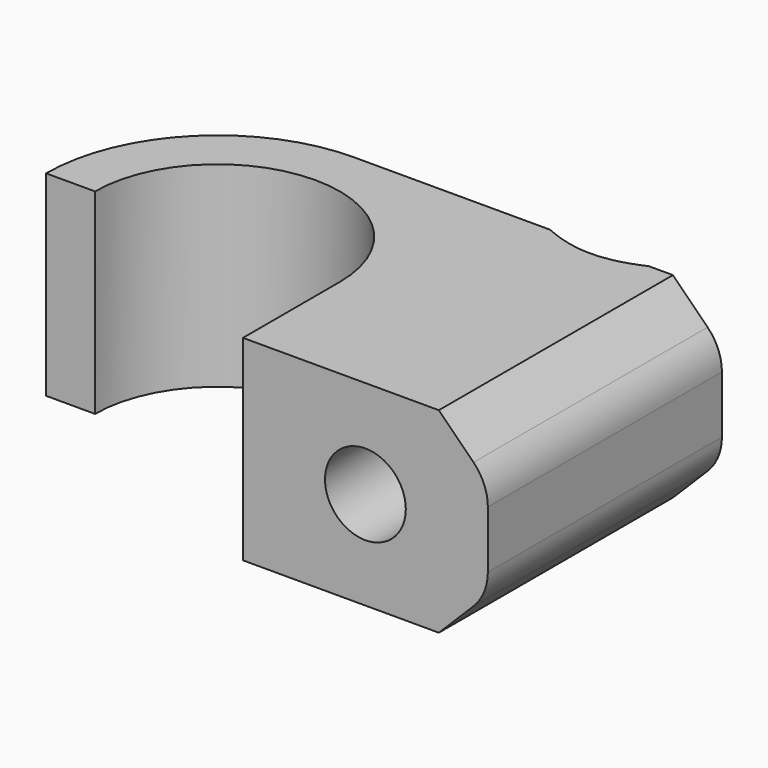
from build123d import *

# Parameters (mm, degrees)
F1_DEPTH       = 4
F3_D           = 3.3
F3_CSINK_D     = 8.96
F3_CSINK_ANGLE = 90
F4_SIZE        = 2
F5_R           = 2


with BuildPart() as f1:
    # F0 (on Top) → F1 (new body, symmetric)
    with BuildSketch(Plane.XY):
        with BuildLine():
            ThreePointArc((-53.8887429237, 51.9443377852), (-48.8887429237, 56.9443377852), (-43.8887429237, 51.9443377852))
            Line((-43.8887429237, 51.9443377852), (-43.8887429237, 46.9949170947))
            Line((-43.8887429237, 46.9949170947), (-33.8887429237, 46.9949170947))
            Line((-33.8887429237, 46.9949170947), (-33.8887429237, 58.9443377852))
            Line((-33.8887429237, 58.9443377852), (-48.8887429237, 58.9443377852))
            ThreePointArc((-48.8887429237, 58.9443377852), (-53.838490392, 56.8940852535), (-55.8887429237, 51.9443377852))
            Line((-55.8887429237, 51.9443377852), (-53.8887429237, 51.9443377852))
        make_face()
    extrude(amount=F1_DEPTH, both=True)

    # F3 (through all)
    with Locations(Plane(origin=(0, 58.9443377852, 0), x_dir=(-1, 0, 0), z_dir=(0, 1, 0))):
        with Locations((38.8887429237, 0)):
            CounterSinkHole(F3_D / 2, F3_CSINK_D / 2, counter_sink_angle=F3_CSINK_ANGLE)

    # F4
    f4_edges = [f1.edges().sort_by_distance(p)[0] for p in [
        (-33.888743, 52.969627, -4),
        (-33.888743, 52.969627, 4),
    ]]
    chamfer(f4_edges, length=F4_SIZE)

    # F5
    f5_edges = [f1.edges().sort_by_distance(p)[0] for p in [
        (-33.888743, 52.969627, 2),
        (-33.888743, 52.969627, -2),
    ]]
    fillet(f5_edges, radius=F5_R)


solid = f1.part
